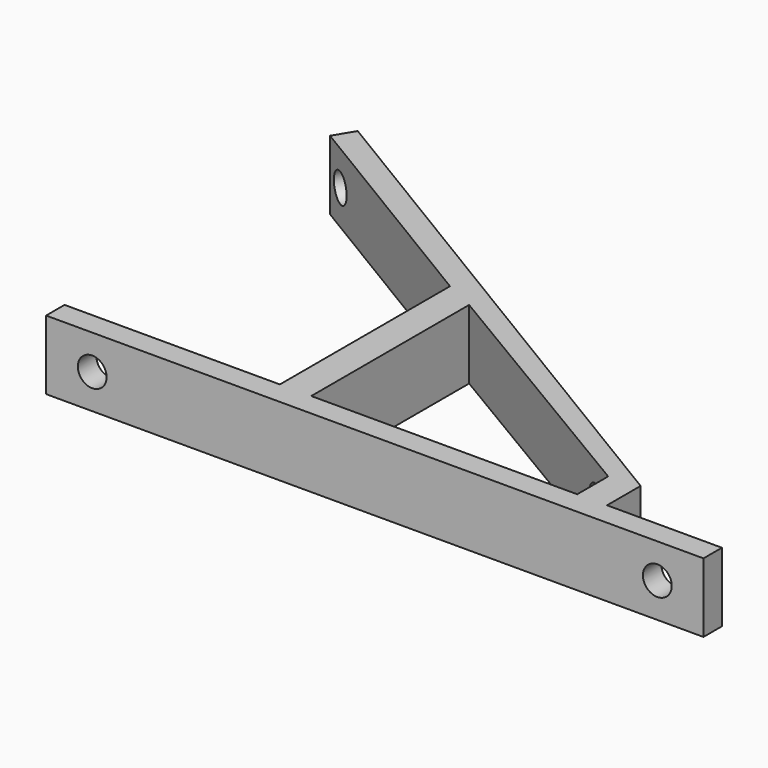
from build123d import *

# Parameters (mm, degrees)
F1_DEPTH = 3
F2_R     = 1.25
F3_DEPTH = 12.5
F4_R     = 1.25
F5_DEPTH = 4


# Not quite as in the source:
# - a feature names something its author has since deleted; it is built from what else it names


with BuildPart() as f1:
    # F0 (on Top) → F1 (new body, symmetric)
    with BuildSketch(Plane.XY):
        Polygon((-38.3288674057, 0), (-57, 0), (-57, -2), (0, -2), (0, 0), (-3.9376540358, 0), (-6.9237630814, 0), (-9.9603020251, 0), (-9.9603020251, 3.6380901354), (-57.4212029734, 32.3077111831), (-58.4553107619, 30.595805496), (-38.3288674057, 18.4380610677), align=None)
        Polygon((-35.6059968472, 0), (-35.6059968472, 17.1079821885), (-12.5451418841, 3.3529622977), (-12.5451418841, 0), align=None, mode=Mode.SUBTRACT)
    extrude(amount=F1_DEPTH, both=True)

    # F2 (on face) → F3 (cut, symmetric)
    with BuildSketch(Plane.XZ.offset(2)):
        with Locations((-53, 0)):
            Circle(F2_R)
        with Locations((-4, 0)):
            Circle(F2_R)
    extrude(amount=F3_DEPTH, both=True, mode=Mode.SUBTRACT)

    # F4 (on face) → F5 (cut)
    with BuildSketch(Plane(origin=(-1.0527110533, -1.7427023171, 0), x_dir=(-0.8559528436, 0.5170538943, 0), z_dir=(0.5170538943, 0.8559528436, 0))):
        with Locations((63.8546698487, 0)):
            Circle(F4_R)
        with Locations((14.8546698487, 0)):
            Circle(F4_R)
    extrude(amount=-F5_DEPTH, mode=Mode.SUBTRACT)


solid = f1.part
